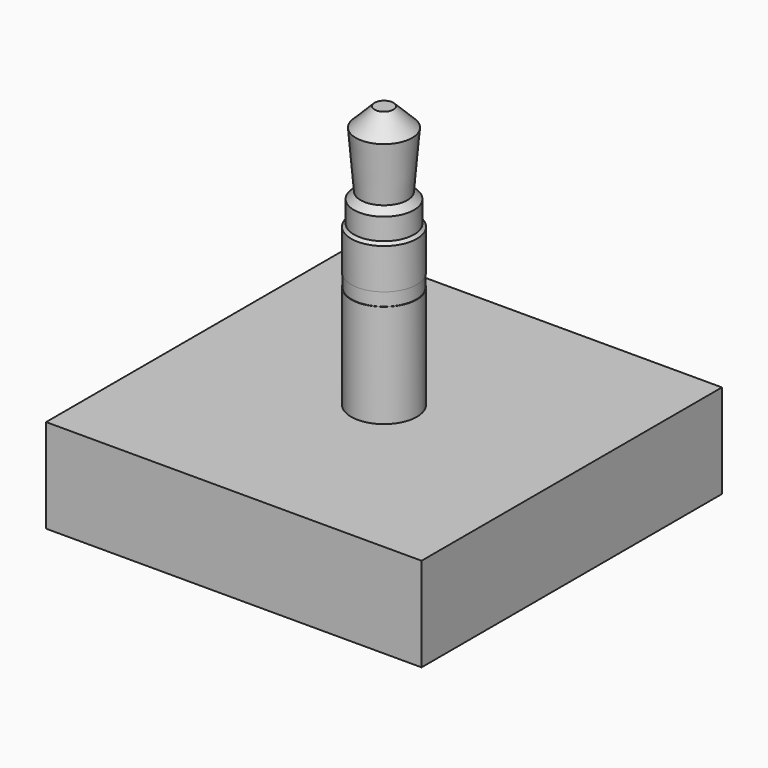
from build123d import *

# Parameters (mm, degrees)
F0_R      = 1.75
F1_DEPTH  = 5.5
F3_R      = 1.725
F4_DEPTH  = 0.7
F6_R      = 1.75
F7_DEPTH  = 2.3
F9_R      = 1.6
F10_DEPTH = 0.7
F12_R     = 1.6
F13_DEPTH = 0.8
F15_R     = 1.25
F17_R     = 1.5
F20_R     = 1.5
F21_DEPTH = 1
F22_SIZE2 = 0.99999
F22_SIZE  = 0.99999
F23_SIZE  = 0.14999
F24_SIZE  = 0.34999
F26_W     = 20
F26_H     = 20
F27_DEPTH = 5


# Not quite as in the source:
# - a fillet or chamfer is up to 0.001 mm smaller than in the source, because OpenCascade refuses the exact size


with BuildPart() as f1:
    # F0 (on Top) → F1 (new body)
    with BuildSketch(Plane.XY):
        Circle(F0_R)
    extrude(amount=F1_DEPTH)

    # F3 (on offset) → F4 (join)
    with BuildSketch(Plane.XY.offset(5.5)):
        Circle(F3_R)
    extrude(amount=F4_DEPTH)

    # F6 (on offset) → F7 (join)
    with BuildSketch(Plane.XY.offset(6.2)):
        Circle(F6_R)
    extrude(amount=F7_DEPTH)

    # F9 (on offset) → F10 (join)
    with BuildSketch(Plane.XY.offset(8.5)):
        Circle(F9_R)
    extrude(amount=F10_DEPTH)

    # F12 (on offset) → F13 (join)
    with BuildSketch(Plane.XY.offset(9.2)):
        Circle(F12_R)
    extrude(amount=F13_DEPTH)

    # F15 (on offset) → F18 section 0
    with BuildSketch(Plane.XY.offset(10)):
        Circle(F15_R)
    # F17 (on offset) → F18 section 1
    with BuildSketch(Plane.XY.offset(13)):
        Circle(F17_R)
    loft()

    # F20 (on offset) → F21 (join)
    with BuildSketch(Plane.XY.offset(13)):
        Circle(F20_R)
    extrude(amount=F21_DEPTH)

    # F22 (size 1 and 1 in the source; OpenCascade refuses exactly that, so slightly less here)
    f22_edges = [f1.edges().sort_by_distance(p)[0] for p in [
        (-1.5, 0, 14),
    ]]
    chamfer(f22_edges, length=F22_SIZE, length2=F22_SIZE2)

    # F23 (size 0.15 in the source; OpenCascade refuses exactly that, so slightly less here)
    f23_edges = [f1.edges().sort_by_distance(p)[0] for p in [
        (-1.75, 0, 8.5),
    ]]
    chamfer(f23_edges, length=F23_SIZE)

    # F24 (size 0.35 in the source; OpenCascade refuses exactly that, so slightly less here)
    f24_edges = [f1.edges().sort_by_distance(p)[0] for p in [
        (-1.6, 0, 10),
    ]]
    chamfer(f24_edges, length=F24_SIZE)

    # F26 (on offset) → F27 (join)
    with BuildSketch(Plane(origin=(0, 0, 0), x_dir=(1, 0, 0), z_dir=(0, 0, -1))):
        Rectangle(F26_W, F26_H)
    extrude(amount=F27_DEPTH)


solid = f1.part
